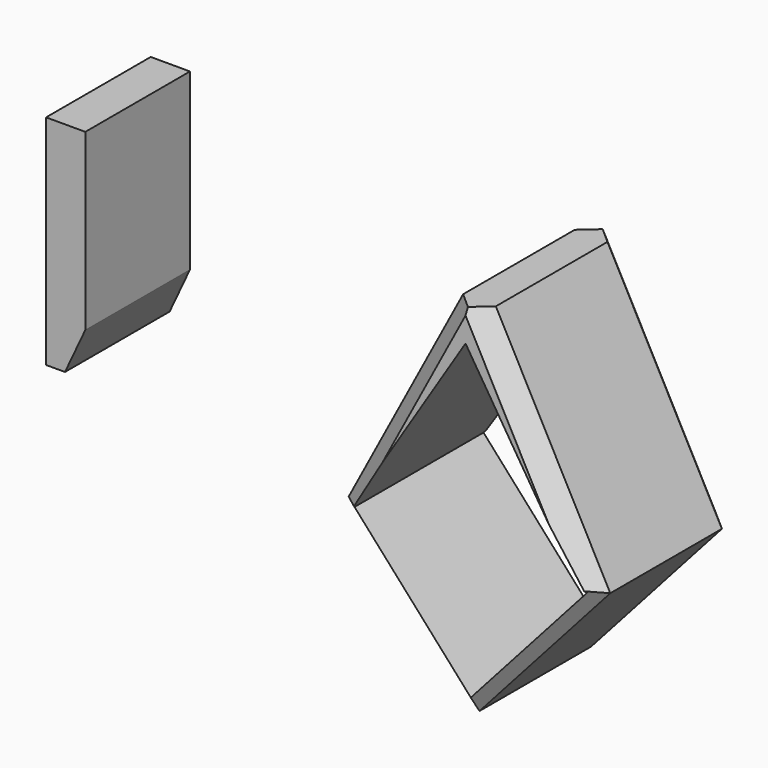
from build123d import *

# Parameters (mm, degrees)
F1_DEPTH    = 50.8
F2_T1_DEPTH = 83.2782991577
F2_T3_DEPTH = 83.2782991577
F2_T5_DEPTH = 107.325076123
F2_T7_DEPTH = 107.325076123
F3_SIZE     = 10.16
F4_W        = 11.43
F4_H        = 63.5
F5_DEPTH    = 38.1
F6_SIZE2    = 5.9221072586
F6_SIZE     = 12.7
F7_W        = 11.43
F7_H        = 63.5
F8_DEPTH    = 50.8
F9_SIZE2    = 13.9571852908
F9_SIZE     = 5.08


# Not quite as in the source:
# - a fillet or chamfer that OpenCascade refuses, or shapes differently, is made with other operations: its cross-section is extruded or revolved along the edge and cut away or added


with BuildPart() as f1:
    # F0 (on Front) → F1 (new body)
    with BuildSketch(Plane.XZ):
        Polygon((38.1, 0), (0, 71.7029050286), (-38.1, 0), (-33.8666666667, 0), (0, 53.7149782546), (33.8666666667, 0), align=None)
        Polygon((0, -42.5970949714), (38.1, 0), (33.8666666667, 0), (0, -37.864084419), (-33.8666666667, 0), (-38.1, 0), align=None)
    extrude(amount=F1_DEPTH)

    # F2: chamfer of 5.08 on 8 edges, made by hand

    # F2_s2 → F2_t1 (cut)
    with BuildSketch(Plane(origin=(-25.6427663859, 0, 28.669484385), x_dir=(0, 1, 0), z_dir=(0.6666666667, 0, -0.7453559925))):
        Polygon((-45.72, -28.3980633142), (-50.8, -23.3180633142), (-50.8, -28.3980633142), align=None)
        Polygon((-5.08, -28.3980633142), (0, -23.3180633142), (0, -28.3980633142), align=None)
    extrude(amount=F2_T1_DEPTH, mode=Mode.SUBTRACT)

    # F2_s4 → F2_t3 (cut)
    with BuildSketch(Plane(origin=(-29.8760997192, 0, -33.4024949374), x_dir=(0, 1, 0), z_dir=(0.6666666667, 0, 0.7453559925))):
        Polygon((-45.72, -28.3980633142), (-50.8, -23.3180633142), (-50.8, -28.3980633142), align=None)
        Polygon((-5.08, -28.3980633142), (0, -23.3180633142), (0, -28.3980633142), align=None)
    extrude(amount=F2_T3_DEPTH, mode=Mode.SUBTRACT)

    # F2_s6 → F2_t5 (cut)
    with BuildSketch(Plane(origin=(35.8413449406, 0, 67.4521929756), x_dir=(0, 1, 0), z_dir=(-0.4692304476, 0, -0.8830757538))):
        Polygon((-45.72, -33.6451862216), (-50.8, -28.5651862216), (-50.8, -33.6451862216), align=None)
        Polygon((-5.08, -33.6451862216), (0, -28.5651862216), (0, -33.6451862216), align=None)
    extrude(amount=F2_T5_DEPTH, mode=Mode.SUBTRACT)

    # F2_s8 → F2_t7 (cut)
    with BuildSketch(Plane(origin=(14.5188485685, 0, -27.3239795285), x_dir=(0, 1, 0), z_dir=(-0.4692304476, 0, 0.8830757538))):
        Polygon((-45.72, -33.6451862216), (-50.8, -28.5651862216), (-50.8, -33.6451862216), align=None)
        Polygon((-5.08, -33.6451862216), (0, -28.5651862216), (0, -33.6451862216), align=None)
    extrude(amount=F2_T7_DEPTH, mode=Mode.SUBTRACT)

    # F3
    f3_edges = [f1.edges().sort_by_distance(p)[0] for p in [
        (0, -25.4, 71.702905),
    ]]
    chamfer(f3_edges, length=F3_SIZE)


with BuildPart() as f5:
    # F4 (on Front) → F5 (new body)
    with BuildSketch(Plane.XZ):
        with Locations((-126.6095284371, 31.75)):
            Rectangle(F4_W, F4_H)
    extrude(amount=F5_DEPTH)

    # F6
    f6_edges = [f5.edges().sort_by_distance(p)[0] for p in [
        (-120.894528, -19.05, 0),
    ]]
    f6_side = f5.faces().sort_by_distance((-120.894528, -19.05, 31.75))[0]
    chamfer(f6_edges, length=F6_SIZE, length2=F6_SIZE2, reference=f6_side)


with BuildPart() as f8:
    # F7 (on Front) → F8 (new body)
    with BuildSketch(Plane.XZ):
        with Locations((127.6592557868, 31.75)):
            Rectangle(F7_W, F7_H)
    extrude(amount=F8_DEPTH)

    # F9
    f9_edges = [f8.edges().sort_by_distance(p)[0] for p in [
        (121.944256, -25.4, 0),
    ]]
    f9_side = f8.faces().sort_by_distance((127.659256, -25.4, 0))[0]
    chamfer(f9_edges, length=F9_SIZE, length2=F9_SIZE2, reference=f9_side)


solid = Compound([f1.part, f5.part])
